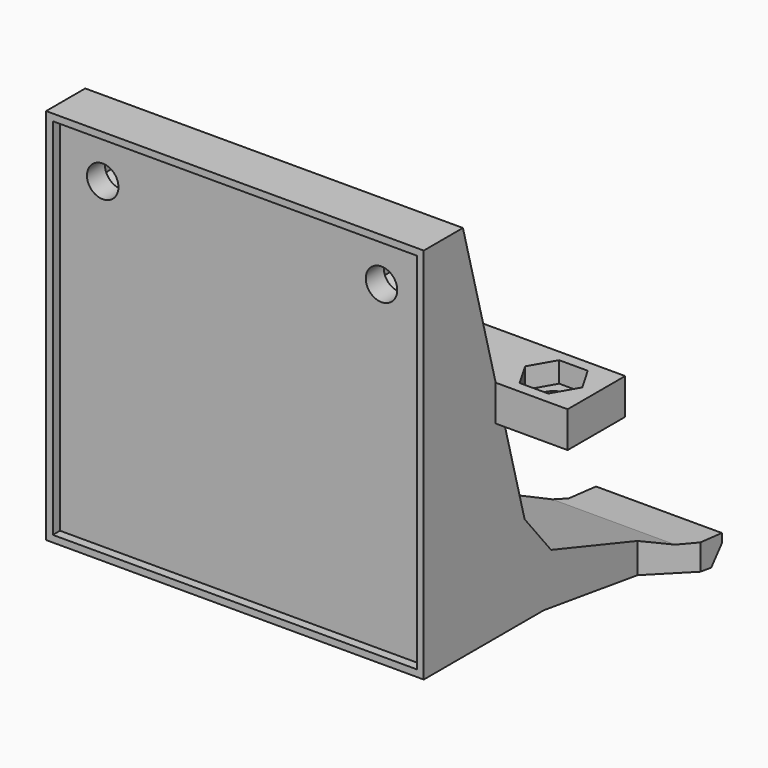
from build123d import *

# Parameters (mm, degrees)
F0_W        = 58
F0_H        = 8
F0_R        = 1.75
F1_DEPTH    = 4
F2_W        = 42
F2_H        = 42
F3_DEPTH    = 10
F5_DEPTH    = 2.3
F7_DEPTH    = 50.001
F9_DEPTH    = 42
F10_R       = 1.75
F11_DEPTH   = 25
F13_DEPTH   = 42
F14_W       = 40.5
F14_H       = 40.5
F15_DEPTH   = 1
F16_SIZE2   = 1.5
F16_SIZE    = 2
F18_DEPTH   = 3
F20_DEPTH   = 3
F21_SIZE2   = 4.99999
F21_SIZE    = 2.99999
F21_2_SIZE2 = 4.99999
F21_2_SIZE  = 2.99999
F24_DEPTH   = 25
F26_DEPTH   = 5


# Not quite as in the source:
# - a fillet or chamfer is up to 0.001 mm smaller than in the source, because OpenCascade refuses the exact size


with BuildPart() as f1:
    # F0 (on Top) → F1 (new body)
    with BuildSketch(Plane.XY):
        Rectangle(F0_W, F0_H)
        with Locations((-24.25, 0)):
            Circle(F0_R, mode=Mode.SUBTRACT)
        with Locations((24.25, 0)):
            Circle(F0_R, mode=Mode.SUBTRACT)
    extrude(amount=F1_DEPTH)

    # F2 (on face) → F3 (join)
    with BuildSketch(Plane.XZ.offset(4)):
        Rectangle(F2_W, F2_H)
    extrude(amount=F3_DEPTH)

    # F4 (on face) → F5 (cut)
    with BuildSketch(Plane.XY.offset(4)):
        Polygon((27.4254264805, 0), (25.8377132403, 2.75), (22.6622867597, 2.75), (21.0745735195, 0), (22.6622867597, -2.75), (25.8377132403, -2.75), align=None)
        Polygon((-22.6622867597, -2.75), (-21.0745735195, 0), (-22.6622867597, 2.75), (-25.8377132403, 2.75), (-27.4254264805, 0), (-25.8377132403, -2.75), align=None)
    extrude(amount=-F5_DEPTH, mode=Mode.SUBTRACT)

    # F6 (on face) → F7 (cut, through all)
    with BuildSketch(Plane(origin=(-21, 0, 0), x_dir=(0, -1, 0), z_dir=(-1, 0, 0))):
        Polygon((8.5551362713, 21), (4, 21), (4, 4), align=None)
    extrude(amount=-F7_DEPTH, mode=Mode.SUBTRACT)

    # F8 (on face) → F9 (join, through all)
    with BuildSketch(Plane(origin=(-21, 0, 0), x_dir=(0, -1, 0), z_dir=(-1, 0, 0))):
        Polygon((4, -21), (4, 0), (2.9282032303, 0), (-2.6987298108, -21), align=None)
    extrude(amount=-F9_DEPTH)

    # F10 (on face) → F11 (cut)
    with BuildSketch(Plane.XZ.offset(14)):
        with Locations((-15.5, 15.5)):
            Circle(F10_R)
        with Locations((15.5, 15.5)):
            Circle(F10_R)
    extrude(amount=-F11_DEPTH, mode=Mode.SUBTRACT)

    # F12 (on face) → F13 (join, through all)
    with BuildSketch(Plane(origin=(-21, 0, 0), x_dir=(0, -1, 0), z_dir=(-1, 0, 0))):
        Polygon((-23.6987298108, -24), (-2.6987298108, -21), (-0.0192378865, -11), (-3.6987298108, -15.5), (-18.6987298108, -20.5), (-23.6987298108, -21), align=None)
    extrude(amount=-F13_DEPTH)

    # F14 (on face) → F15 (cut)
    with BuildSketch(Plane.XZ.offset(14)):
        Rectangle(F14_W, F14_H)
    extrude(amount=-F15_DEPTH, mode=Mode.SUBTRACT)

    # F16
    f16_edges = [f1.edges().sort_by_distance(p)[0] for p in [
        (0, 23.69873, -24),
    ]]
    f16_side = f1.faces().sort_by_distance((0, 23.69873, -22.5))[0]
    chamfer(f16_edges, length=F16_SIZE, length2=F16_SIZE2, reference=f16_side)

    # F17 (on face) → F18 (join)
    with BuildSketch(Plane(origin=(-21, 0, 0), x_dir=(0, -1, 0), z_dir=(-1, 0, 0))):
        Polygon((-23.6987298108, -21), (-23.6987298108, -22), (-22.2138055703, -23.7878679656), (-15.6987298108, -22.8571428571), (-15.6987298108, -19.5), (-18.6987298108, -20.5), align=None)
    extrude(amount=F18_DEPTH)

    # F19 (on face) → F20 (join)
    with BuildSketch(Plane.YZ.offset(21)):
        Polygon((15.6987298108, -22.8571428571), (22.2138055703, -23.7878679656), (23.6987298108, -22), (23.6987298108, -21), (18.6987298108, -20.5), (15.6987298108, -19.5), align=None)
    extrude(amount=F20_DEPTH)

    # F21 (size 3 and 5 in the source; OpenCascade refuses exactly that, so slightly less here)
    f21_edges = [f1.edges().sort_by_distance(p)[0] for p in [
        (24, 15.69873, -21.178571),
    ]]
    f21_side = f1.faces().sort_by_distance((22.5, 15.69873, -21.178571))[0]
    chamfer(f21_edges, length=F21_SIZE, length2=F21_SIZE2, reference=f21_side)

    # F21#2 (size 3 and 5 in the source; OpenCascade refuses exactly that, so slightly less here)
    f21_2_edges = [f1.edges().sort_by_distance(p)[0] for p in [
        (-24, 15.69873, -21.178571),
    ]]
    f21_2_side = f1.faces().sort_by_distance((-22.5, 15.69873, -21.178571))[0]
    chamfer(f21_2_edges, length=F21_2_SIZE, length2=F21_2_SIZE2, reference=f21_2_side)

    # F23 (on offset) → F24 (cut)
    with BuildSketch(Plane.XZ.offset(10.5)):
        Polygon((12.75, 17.0877132403), (12.75, 13.9122867597), (15.5, 12.3245735195), (18.25, 13.9122867597), (18.25, 17.0877132403), (15.5, 18.6754264805), align=None)
        Polygon((-12.75, 13.9122867597), (-12.75, 17.0877132403), (-15.5, 18.6754264805), (-18.25, 17.0877132403), (-18.25, 13.9122867597), (-15.5, 12.3245735195), align=None)
    extrude(amount=-F24_DEPTH, mode=Mode.SUBTRACT)

    # F25 (on face) → F26 (cut, symmetric)
    with BuildSketch(Plane(origin=(0, 0, -21), x_dir=(1, 0, 0), z_dir=(0, 0, -1))):
        Polygon((-10, -23.6987298108), (10, -23.6987298108), (10, -19.9001319306), (0, -5.6186518632), (-10, -19.9001319306), align=None)
    extrude(amount=F26_DEPTH, both=True, mode=Mode.SUBTRACT)


solid = f1.part
